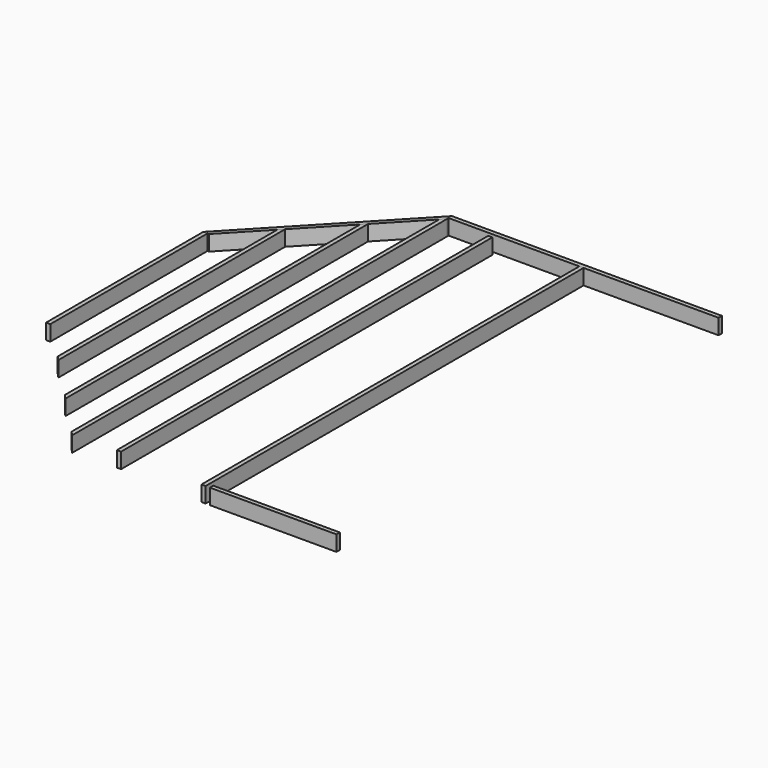
from build123d import *

# Parameters (mm, degrees)
F1_DEPTH = 69.85
F0_W     = 38.1
F0_H     = 4191
F0_H_2   = 1773.8625425149
F2_DEPTH = 69.85
F3_DEPTH = 69.85


with BuildPart() as f1:
    # F0 (on Top) → F1 (new body, symmetric)
    with BuildSketch(Plane.XY):
        Polygon((0, 0), (0, 2133.6), (-38.1, 2133.6), (-38.1, 2095.5), (-38.1, -2095.5), (-38.1, -2133.6), (0, -2133.6), align=None)
    extrude(amount=F1_DEPTH, both=True)


with BuildPart() as f1b:
    # F0 (on Top) → F1, piece 2 (new body, symmetric)
    with BuildSketch(Plane.XY):
        Polygon((387.35, -2095.5), (38.1, -2095.5), (38.1, -2133.6), (1181.1, -2133.6), (1181.1, -2095.5), (831.85, -2095.5), (793.75, -2095.5), (425.45, -2095.5), align=None)
    extrude(amount=F1_DEPTH, both=True)


with BuildPart() as f1c:
    # F0 (on Top) → F1, piece 3 (new body, symmetric)
    with BuildSketch(Plane.XY):
        Polygon((-1219.2, -2116.3506185252), (-1219.2, 2116.3506185252), (-1257.3, 2076.201595752), (-1257.3, -2076.201595752), align=None)
    extrude(amount=F1_DEPTH, both=True)


with BuildPart() as f1d:
    # F0 (on Top) → F1, piece 4 (new body, symmetric)
    with BuildSketch(Plane.XY):
        with Locations((-812.8, 0)):
            Rectangle(F0_W, F0_H)
    extrude(amount=F1_DEPTH, both=True)


with BuildPart() as f1e:
    # F0 (on Top) → F1, piece 5 (new body, symmetric)
    with BuildSketch(Plane.XY):
        with Locations((-2419.35, 0)):
            Rectangle(F0_W, F0_H_2)
    extrude(amount=F1_DEPTH, both=True)


with BuildPart() as f1f:
    # F0 (on Top) → F1, piece 6 (new body, symmetric)
    with BuildSketch(Plane.XY):
        Polygon((-1606.55, -1708.1688869976), (-1606.55, 1708.1688869976), (-1644.65, 1668.0198642244), (-1644.65, -1668.0198642244), align=None)
    extrude(amount=F1_DEPTH, both=True)


with BuildPart() as f1g:
    # F0 (on Top) → F1, piece 7 (new body, symmetric)
    with BuildSketch(Plane.XY):
        Polygon((-2012.95, 1279.9126440834), (-2051.05, 1239.7636213102), (-2051.05, -1239.7636213102), (-2012.95, -1279.9126440834), align=None)
    extrude(amount=F1_DEPTH, both=True)


with BuildPart() as f2:
    # F0 (on Top) → F2 (new body, symmetric)
    with BuildSketch(Plane.XY):
        Polygon((0, 2133.6), (38.1, 2133.6), (1181.1, 2133.6), (1219.2, 2133.6), (1219.2, 2171.7), (-1219.2, 2171.7), (-1219.2, 2133.6), (-1181.1, 2133.6), (-38.1, 2133.6), align=None)
    extrude(amount=F2_DEPTH, both=True)


with BuildPart() as f3:
    # F0 (on Top) → F3 (new body, symmetric)
    with BuildSketch(Plane.XY):
        Polygon((-1219.2, 2116.3506185252), (-1219.2, 2133.6), (-1219.2, 2171.7), (-2438.4, 886.9312712575), (-2400.3, 886.9312712575), (-2385.8753981908, 886.9312712575), (-2051.05, 1239.7636213102), (-2012.95, 1279.9126440834), (-1644.65, 1668.0198642244), (-1606.55, 1708.1688869976), (-1257.3, 2076.201595752), align=None)
    extrude(amount=F3_DEPTH, both=True)


solid = Compound([f1.part, f1b.part, f1c.part, f1d.part, f1e.part, f1f.part, f1g.part, f2.part, f3.part])
